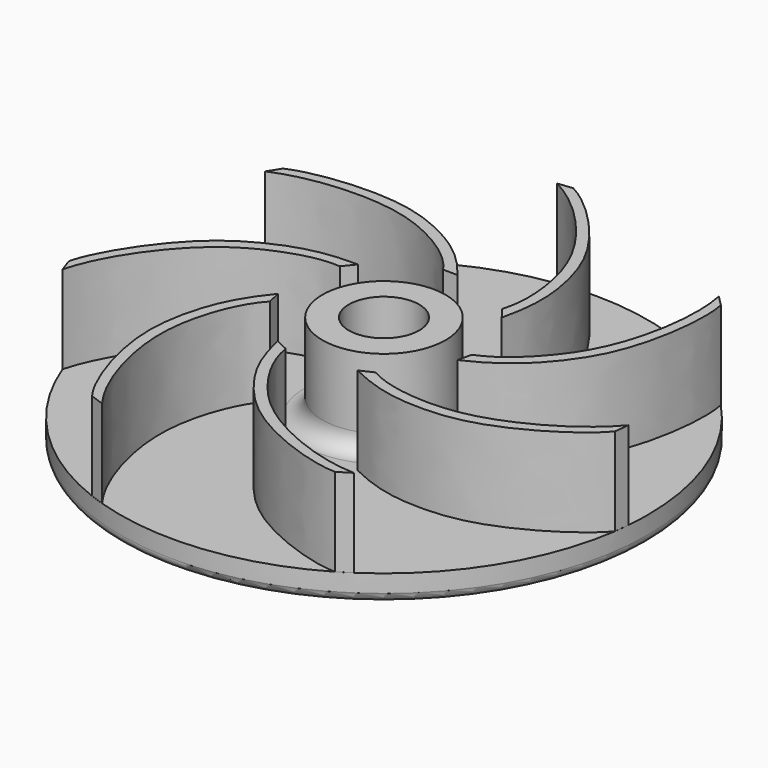
from build123d import *

# Parameters (mm, degrees)
F0_R     = 30
F1_DEPTH = 3
F3_DEPTH = 10
F5_COUNT = 7
F6_R     = 7
F7_DEPTH = 10
F8_R     = 4
F9_DEPTH = 13.001
F10_R    = 1
F11_R    = 2


with BuildPart() as f1:
    # F0 (on Top) → F1 (new body)
    with BuildSketch(Plane.XY):
        Circle(F0_R)
    extrude(amount=F1_DEPTH)

    # F2 (on face) → F3 (join)
    with BuildSketch(Plane.XY.offset(3)):
        with BuildLine():
            Line((-1.6446796944, 10.4644708335), (0, 10.4520414025))
            add(Edge.make_bspline(
                [(0, 10.4520414025), (-2.2289291518, 13.3403059975), (-6.1904321331, 16.1620932905), (-13.6442423507, 18.8532101818), (-22.3243720829, 17.9140381515), (-24.8817240251, 16.7600659168)],
                knots=[0, 0, 0, 0, 0.3225761243, 0.6326131084, 1, 1, 1, 1], degree=3))
            Line((-24.8817240251, 16.7600659168), (-25.7866161055, 15.3313544682))
            add(Edge.make_bspline(
                [(-1.6446796944, 10.4644708335), (-2.8414923982, 12.2416667658), (-7.1707724103, 15.3826694675), (-14.4971888519, 17.5675164501), (-22.4425556004, 16.8143108506), (-25.7866161055, 15.3313544682)],
                knots=[0, 0, 0, 0, 0.3011184154, 0.6179723344, 1, 1, 1, 1], degree=3))
        make_face()
    extrude(amount=F3_DEPTH)


with BuildPart() as f5_1:
    # F5: instance of F1
    add(f1.part.rotate(Axis((0, 0, 22.8564720601), (0, 0, 1)), 1 * 360 / F5_COUNT))


with BuildPart() as f5_2:
    # F5: instance of F1
    add(f1.part.rotate(Axis((0, 0, 22.8564720601), (0, 0, 1)), 2 * 360 / F5_COUNT))


with BuildPart() as f5_3:
    # F5: instance of F1
    add(f1.part.rotate(Axis((0, 0, 22.8564720601), (0, 0, 1)), 3 * 360 / F5_COUNT))


with BuildPart() as f5_4:
    # F5: instance of F1
    add(f1.part.rotate(Axis((0, 0, 22.8564720601), (0, 0, 1)), 4 * 360 / F5_COUNT))


with BuildPart() as f5_5:
    # F5: instance of F1
    add(f1.part.rotate(Axis((0, 0, 22.8564720601), (0, 0, 1)), 5 * 360 / F5_COUNT))


with BuildPart() as f5_6:
    # F5: instance of F1
    add(f1.part.rotate(Axis((0, 0, 22.8564720601), (0, 0, 1)), 6 * 360 / F5_COUNT))


with BuildPart() as f1_1:
    add(f1.part)

    add(f5_1.part)  # F7 merges F5_1

    add(f5_2.part)  # F7 merges F5_2

    add(f5_3.part)  # F7 merges F5_3

    add(f5_4.part)  # F7 merges F5_4

    add(f5_5.part)  # F7 merges F5_5

    add(f5_6.part)  # F7 merges F5_6
    # F6 (on face) → F7 (join)
    with BuildSketch(Plane.XY.offset(3)):
        Circle(F6_R)
    extrude(amount=F7_DEPTH)

    # F8 (on face) → F9 (cut, through all)
    with BuildSketch(Plane.XY.offset(13)):
        Circle(F8_R)
    extrude(amount=-F9_DEPTH, mode=Mode.SUBTRACT)

    # F10
    f10_edges = [f1_1.edges().sort_by_distance(p)[0] for p in [
        (-18.704694, 23.454944, 0),
    ]]
    fillet(f10_edges, radius=F10_R)

    # F11
    f11_edges = [f1_1.edges().sort_by_distance(p)[0] for p in [
        (-7, 0, 3),
    ]]
    fillet(f11_edges, radius=F11_R)


solid = f1_1.part
